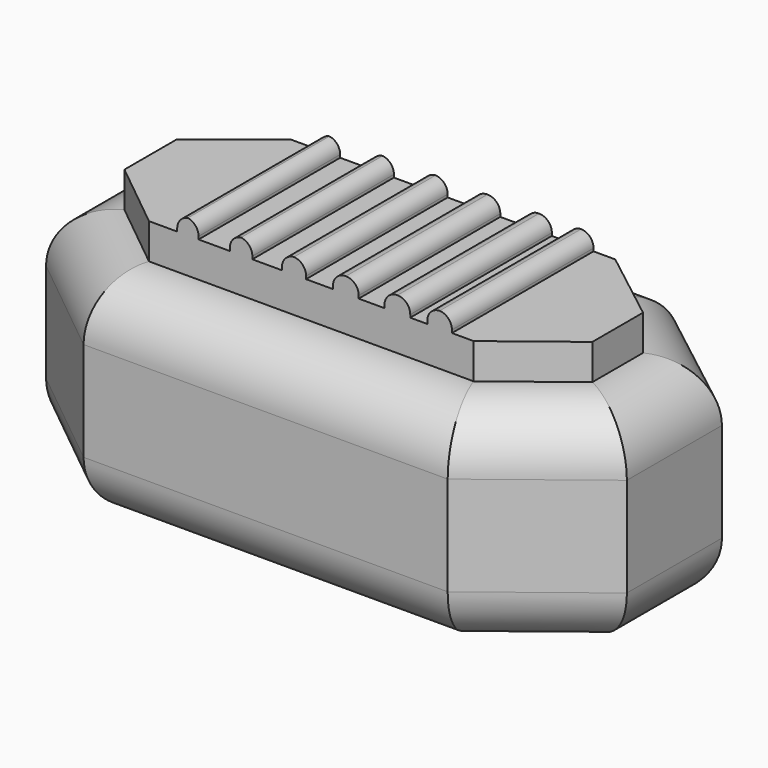
from build123d import *

# Parameters (mm, degrees)
F1_DEPTH    = 38.1
F2_R        = 10.16
F3_R        = 10.16
F5_DEPTH    = 6.35
F6_W        = 3.8326773793
F6_H        = 31.7183228926
F6_W_2      = 4.029225558
F6_W_3      = 4.3240477098
F6_W_4      = 4.6188691631
F6_W_5      = 4.6188682318
F6_W_6      = 4.4223219156
F7_DEPTH    = 2.794
F8_T1_DEPTH = 43.1483228926


# Not quite as in the source:
# - a fillet or chamfer that OpenCascade refuses, or shapes differently, is made with other operations: its cross-section is extruded or revolved along the edge and cut away or added


with BuildPart() as f1:
    # F0 (on Top) → F1 (new body)
    with BuildSketch(Plane.XY):
        Polygon((-33.02, -26.0191614463), (32.2342477739, -26.0191614463), (52.0383228926, -10.6488130987), (52.0383228926, 10.6521614463), (32.2342477739, 26.0191614463), (-33.02, 26.0191614463), (-52.0383228926, 10.6521614463), (-52.0383228926, -10.6488130987), align=None)
    extrude(amount=F1_DEPTH)

    # F2
    f2_edges = [f1.edges().sort_by_distance(p)[0] for p in [
        (-0.392876, -26.019161, 38.1),
        (-42.529161, -18.333987, 38.1),
        (-52.038323, 0.001674, 38.1),
        (-42.529161, 18.335661, 38.1),
        (-0.392876, 26.019161, 38.1),
        (42.136285, 18.335661, 38.1),
        (52.038323, 0.001674, 38.1),
        (42.136285, -18.333987, 38.1),
    ]]
    fillet(f2_edges, radius=F2_R)

    # F3
    f3_edges = [f1.edges().sort_by_distance(p)[0] for p in [
        (-0.392876, -26.019161, 0),
        (-42.529161, -18.333987, 0),
        (-52.038323, 0.001674, 0),
        (-42.529161, 18.335661, 0),
        (-0.392876, 26.019161, 0),
        (42.136285, 18.335661, 0),
        (52.038323, 0.001674, 0),
        (42.136285, -18.333987, 0),
    ]]
    fillet(f3_edges, radius=F3_R)

    # F4 (on face) → F5 (join)
    with BuildSketch(Plane.XY.offset(38.1)):
        Polygon((-29.4282840059, 15.8591614463), (-41.8783228926, 5.7994023049), (-41.8783228926, -5.7967184312), (-29.4276753196, -15.8591614463), (28.7541399654, -15.8591614463), (41.8783228926, -5.6732142531), (41.8783228926, 5.6758979589), (28.7547389102, 15.8591614463), align=None)
    extrude(amount=F5_DEPTH)

    # F6 (on face) → F7 (join)
    with BuildSketch(Plane.XY.offset(44.45)):
        with Locations((-22.4555665627, 0)):
            Rectangle(F6_W, F6_H)
        with Locations((-12.9230059683, 0)):
            Rectangle(F6_W_2, F6_H)
        with Locations((-3.4395834082, 0)):
            Rectangle(F6_W_3, F6_H)
        with Locations((5.8472915553, 0)):
            Rectangle(F6_W_4, F6_H)
        with Locations((15.0850303471, 0)):
            Rectangle(F6_W_5, F6_H)
        with Locations((22.6521138102, 0)):
            Rectangle(F6_W_6, F6_H)
    extrude(amount=F7_DEPTH)

    # F8: fillet of radius 2.286 on 12 edges, made by hand

    # F8_s2 → F8_t1 (cut)
    with BuildSketch(Plane.XZ.offset(-21.5741614463)):
        with BuildLine():
            ThreePointArc((-20.5392278731, 44.958), (-21.2087817713, 46.5744461018), (-22.8252278731, 47.244))
            Line((-22.8252278731, 47.244), (-20.5392278731, 47.244))
            Line((-20.5392278731, 47.244), (-20.5392278731, 44.958))
        make_face()
        with BuildLine():
            ThreePointArc((-10.9083931893, 44.958), (-11.5779470875, 46.5744461018), (-13.1943931893, 47.244))
            Line((-13.1943931893, 47.244), (-10.9083931893, 47.244))
            Line((-10.9083931893, 47.244), (-10.9083931893, 44.958))
        make_face()
        with BuildLine():
            ThreePointArc((-1.2775595533, 44.958), (-1.9471134515, 46.5744461018), (-3.5635595533, 47.244))
            Line((-3.5635595533, 47.244), (-1.2775595533, 47.244))
            Line((-1.2775595533, 47.244), (-1.2775595533, 44.958))
        make_face()
        with BuildLine():
            ThreePointArc((8.1567261368, 44.958), (7.4871722386, 46.5744461018), (5.8707261368, 47.244))
            Line((5.8707261368, 47.244), (8.1567261368, 47.244))
            Line((8.1567261368, 47.244), (8.1567261368, 44.958))
        make_face()
        with BuildLine():
            ThreePointArc((17.394464463, 44.958), (16.7249105648, 46.5744461018), (15.108464463, 47.244))
            Line((15.108464463, 47.244), (17.394464463, 47.244))
            Line((17.394464463, 47.244), (17.394464463, 44.958))
        make_face()
        with BuildLine():
            ThreePointArc((24.863274768, 44.958), (24.1937208698, 46.5744461018), (22.577274768, 47.244))
            Line((22.577274768, 47.244), (24.863274768, 47.244))
            Line((24.863274768, 47.244), (24.863274768, 44.958))
        make_face()
        with BuildLine():
            ThreePointArc((20.4409528524, 44.958), (21.1105067506, 46.5744461018), (22.7269528524, 47.244))
            Line((22.7269528524, 47.244), (20.4409528524, 47.244))
            Line((20.4409528524, 47.244), (20.4409528524, 44.958))
        make_face()
        with BuildLine():
            ThreePointArc((12.7755962312, 44.958), (13.4451501294, 46.5744461018), (15.0615962312, 47.244))
            Line((15.0615962312, 47.244), (12.7755962312, 47.244))
            Line((12.7755962312, 47.244), (12.7755962312, 44.958))
        make_face()
        with BuildLine():
            ThreePointArc((3.5378569737, 44.958), (4.2074108719, 46.5744461018), (5.8238569737, 47.244))
            Line((5.8238569737, 47.244), (3.5378569737, 47.244))
            Line((3.5378569737, 47.244), (3.5378569737, 44.958))
        make_face()
        with BuildLine():
            ThreePointArc((-5.6016072631, 44.958), (-4.9320533649, 46.5744461018), (-3.3156072631, 47.244))
            Line((-3.3156072631, 47.244), (-5.6016072631, 47.244))
            Line((-5.6016072631, 47.244), (-5.6016072631, 44.958))
        make_face()
        with BuildLine():
            ThreePointArc((-14.9376187474, 44.958), (-14.2680648491, 46.5744461018), (-12.6516187474, 47.244))
            Line((-12.6516187474, 47.244), (-14.9376187474, 47.244))
            Line((-14.9376187474, 47.244), (-14.9376187474, 44.958))
        make_face()
        with BuildLine():
            ThreePointArc((-24.3719052523, 44.958), (-23.7023513541, 46.5744461018), (-22.0859052523, 47.244))
            Line((-22.0859052523, 47.244), (-24.3719052523, 47.244))
            Line((-24.3719052523, 47.244), (-24.3719052523, 44.958))
        make_face()
    extrude(amount=F8_T1_DEPTH, mode=Mode.SUBTRACT)


solid = f1.part
